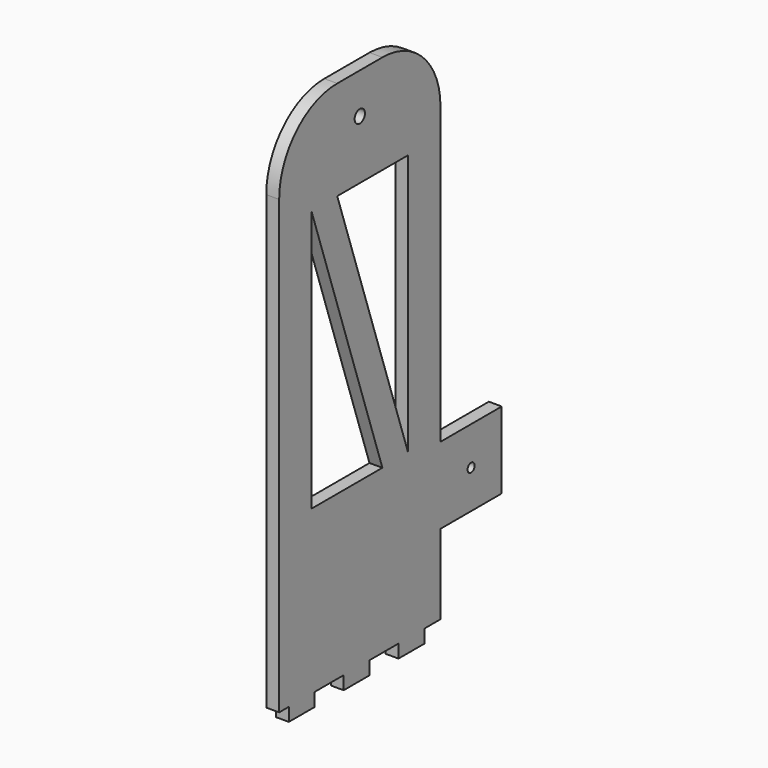
from build123d import *

# Parameters (mm, degrees)
F0_R     = 1.6
F0_W     = 8
F0_H     = 3.3
F0_W_2   = 19
F0_H_2   = 19
F0_R_2   = 1.1
F1_DEPTH = 3.2


# Not quite as in the source:
# - a feature names something its author has since deleted; it is built from what else it names


with BuildPart() as f1:
    # F0 (on Right) → F1 (new body)
    with BuildSketch(Plane.YZ):
        with BuildLine():
            ThreePointArc((-16.7558317706, 130), (-29.483753832, 124.7279220614), (-34.7558317706, 112))
            Line((-34.7558317706, 112), (-34.7558317706, 0))
            Line((-34.7558317706, 0), (-31.7558317706, 0))
            Line((-31.7558317706, 0), (-23.7558317706, 0))
            Line((-23.7558317706, 0), (-14.7558317706, 0))
            Line((-14.7558317706, 0), (-6.7558317706, 0))
            Line((-6.7558317706, 0), (2.2441682294, 0))
            Line((2.2441682294, 0), (10.2441682294, 0))
            Line((10.2441682294, 0), (15.2441682294, 0))
            Line((15.2441682294, 0), (15.2441682294, 19.74954395))
            Line((15.2441682294, 19.74954395), (15.2441682294, 38.74954395))
            Line((15.2441682294, 38.74954395), (15.2441682294, 112))
            ThreePointArc((15.2441682294, 112), (9.9720902908, 124.7279220614), (-2.7558317706, 130))
            Line((-2.7558317706, 130), (-16.7558317706, 130))
        make_face()
        Polygon((-24.7558317706, 40.4), (-24.7558317706, 105.4), (-16.7558317706, 105.4), (5.2441682294, 105.4), (5.2441682294, 40.4), (-2.7558317706, 40.4), align=None, mode=Mode.SUBTRACT)
        with Locations((-9.7558317706, 120)):
            Circle(F0_R, mode=Mode.SUBTRACT)
        with Locations((-27.7558317706, -1.65)):
            Rectangle(F0_W, F0_H)
        with Locations((-10.7558317706, -1.65)):
            Rectangle(F0_W, F0_H)
        with Locations((24.7441682294, 29.24954395)):
            Rectangle(F0_W_2, F0_H_2)
        with Locations((24.7441682294, 29.24954395)):
            Circle(F0_R_2, mode=Mode.SUBTRACT)
        with Locations((6.2441682294, -1.65)):
            Rectangle(F0_W, F0_H)
        Polygon((-16.7558317706, 105.4), (-24.7558317706, 105.4), (-2.7558317706, 40.4), (5.2441682294, 40.4), align=None)
    extrude(amount=F1_DEPTH)


solid = f1.part
